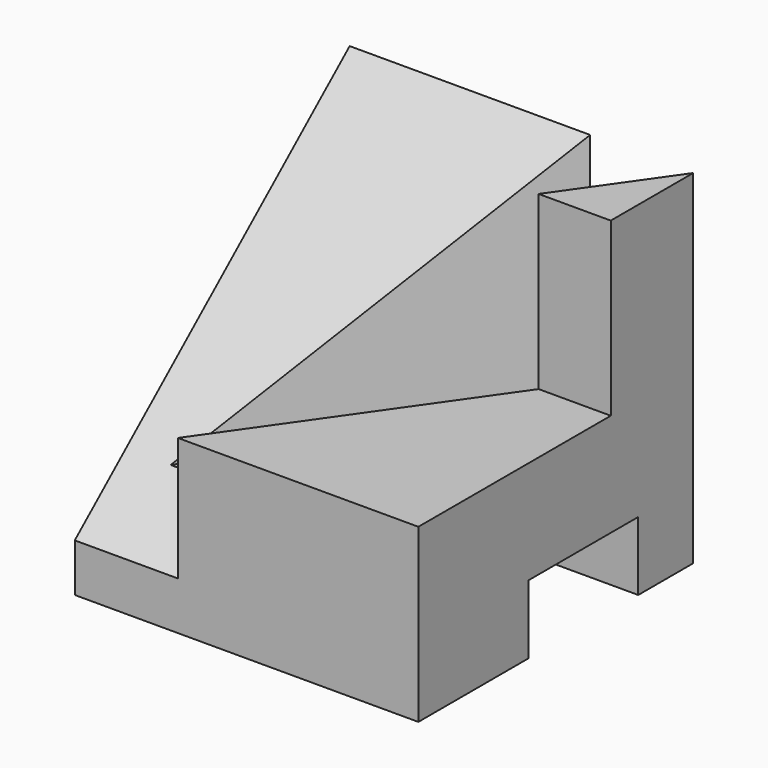
from build123d import *

# Parameters (mm, degrees)
F0_W      = 50
F0_H      = 50
F1_DEPTH  = 50
F2_W      = 20
F2_H      = 10
F3_DEPTH  = 30
F8_DEPTH  = 35
F10_DEPTH = 25
F12_REACH = 115.9479483752


with BuildPart() as f1:
    # F0 (on Top) → F1 (new body)
    with BuildSketch(Plane.XY):
        with Locations((25, 25)):
            Rectangle(F0_W, F0_H)
    extrude(amount=F1_DEPTH)

    # F2 (on face) → F3 (cut)
    with BuildSketch(Plane.YZ.offset(50)):
        with Locations((30, 5)):
            Rectangle(F2_W, F2_H)
    extrude(amount=-F3_DEPTH, mode=Mode.SUBTRACT)

    # F7 (on face) → F8 (cut)
    with BuildSketch(Plane.XY.offset(50)):
        Polygon((15, 0), (50, 50), (35, 50), (0, 0), align=None)
    extrude(amount=-F8_DEPTH, mode=Mode.SUBTRACT)

    # F9 (on face) → F10 (cut)
    with BuildSketch(Plane.XY.offset(50)):
        Polygon((15, 0), (50, 0), (50, 35), (39.5, 35), align=None)
    extrude(amount=-F10_DEPTH, mode=Mode.SUBTRACT)

    f12_end = Plane(origin=(37.75, 32.5, 27.5), x_dir=(-0.5734623444, -0.8192319205, 0), z_dir=(-0.8192319205, 0.5734623444, 0))
    # F11 (on face) → F12 (cut, up to a plane its end follows)
    with BuildSketch(Plane(origin=(0, 0, 0), x_dir=(0, -1, 0), z_dir=(-1, 0, 0))):
        Polygon((0, 50), (-50, 50), (0, 7), align=None)
    f12_long = extrude(amount=-F12_REACH, mode=Mode.PRIVATE)
    add(split(f12_long, bisect_by=f12_end, keep=Keep.TOP, mode=Mode.PRIVATE), mode=Mode.SUBTRACT)


solid = f1.part
